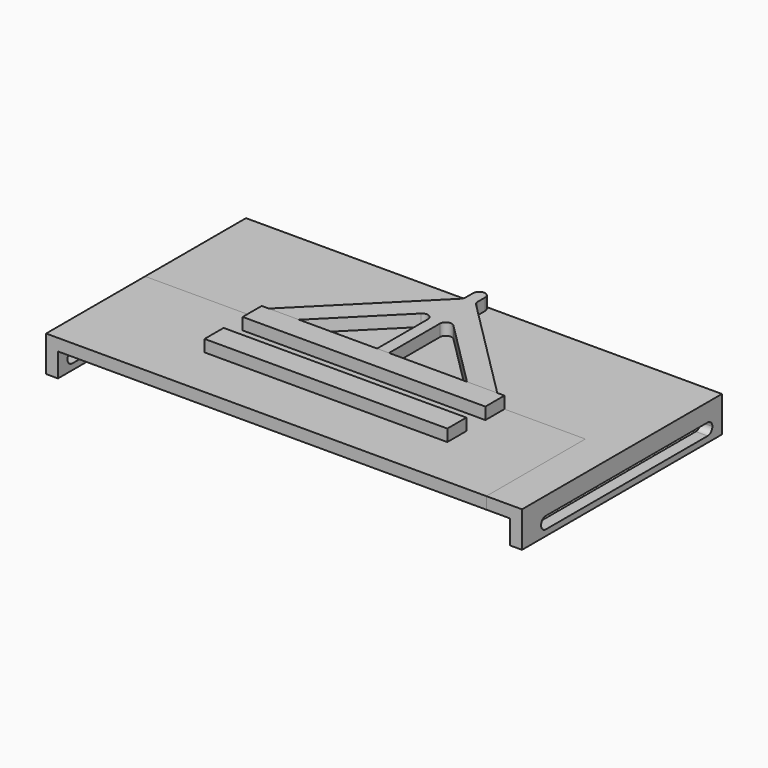
from build123d import *

# Parameters (mm, degrees)
F0_W      = 5
F0_H      = 53
F0_W_2    = 10
F0_H_2    = 10
F1_DEPTH  = 5
F2_DEPTH  = 10
F3_DEPTH  = 10
F0_W_3    = 48.5
F4_DEPTH  = 5
F5_DEPTH  = 10
F6_DEPTH  = 10
F8_DEPTH  = 25
F10_DEPTH = 25


with BuildPart() as f1:
    # F0 (on Top) → F1 (new body)
    with BuildSketch(Plane.XY):
        with Locations((97.5, 26)):
            Rectangle(F0_W, F0_H)
        with BuildLine():
            Line((0, 52.5), (-100, 52.5))
            Line((-100, 52.5), (-100, -0.5))
            Line((-100, -0.5), (-95, -0.5))
            Line((-95, -0.5), (-51, -0.5))
            Line((-51, -0.5), (-48, -0.5))
            Line((-48, -0.5), (-3.232233047, 44.267766953))
            ThreePointArc((-3.232233047, 44.267766953), (-2.6903011687, 45.078825325), (-2.5, 46.0355339059))
            Line((-2.5, 46.0355339059), (-2.5, 50))
            ThreePointArc((-2.5, 50), (-1.767766953, 51.767766953), (0, 52.5))
        make_face()
        with BuildLine():
            Line((85, 52.5), (0, 52.5))
            ThreePointArc((0, 52.5), (1.767766953, 51.767766953), (2.5, 50))
            Line((2.5, 50), (2.5, 46.0355339059))
            ThreePointArc((2.5, 46.0355339059), (2.6903011687, 45.078825325), (3.232233047, 44.267766953))
            Line((3.232233047, 44.267766953), (48, -0.5))
            Line((48, -0.5), (51, -0.5))
            Line((51, -0.5), (85, -0.5))
            Line((85, -0.5), (85, 52.5))
        make_face()
        with BuildLine():
            ThreePointArc((2.5, 50), (1.767766953, 51.767766953), (0, 52.5))
            ThreePointArc((0, 52.5), (-1.767766953, 51.767766953), (-2.5, 50))
            Line((-2.5, 50), (-2.5, 46.0355339059))
            Line((-2.5, 46.0355339059), (-2.5, 32.2720779386))
            Line((-2.5, 32.2720779386), (-2.5, 26.2365440327))
            Line((-2.5, 26.2365440327), (-2.5, 0))
            Line((-2.5, 0), (-2.5, -0.5))
            Line((-2.5, -0.5), (2.5, -0.5))
            Line((2.5, -0.5), (2.5, 26.2365440327))
            Line((2.5, 26.2365440327), (2.5, 46.0355339059))
            Line((2.5, 46.0355339059), (2.5, 50))
        make_face()
        with BuildLine():
            Line((-2.5, 32.2720779386), (-2.5, 46.0355339059))
            ThreePointArc((-2.5, 46.0355339059), (-2.6903011687, 45.078825325), (-3.232233047, 44.267766953))
            Line((-3.232233047, 44.267766953), (-48, -0.5))
            Line((-48, -0.5), (-35.2720779386, -0.5))
            Line((-35.2720779386, -0.5), (-6.767766953, 28.0043109857))
            ThreePointArc((-6.767766953, 28.0043109857), (-4.0432914191, 28.546242864), (-2.5, 26.2365440327))
            Line((-2.5, 26.2365440327), (-2.5, 32.2720779386))
        make_face()
        with BuildLine():
            Line((-2.5, 0), (-2.5, 26.2365440327))
            ThreePointArc((-2.5, 26.2365440327), (-4.0432914191, 28.546242864), (-6.767766953, 28.0043109857))
            Line((-6.767766953, 28.0043109857), (-35.2720779386, -0.5))
            Line((-35.2720779386, -0.5), (-2.5, -0.5))
            Line((-2.5, -0.5), (-2.5, 0))
        make_face()
        with BuildLine():
            ThreePointArc((6.767766953, 28.0043109857), (4.0432914191, 28.546242864), (2.5, 26.2365440327))
            Line((2.5, 26.2365440327), (2.5, -0.5))
            Line((2.5, -0.5), (35.2720779386, -0.5))
            Line((35.2720779386, -0.5), (6.767766953, 28.0043109857))
        make_face()
        with BuildLine():
            ThreePointArc((3.232233047, 44.267766953), (2.6903011687, 45.078825325), (2.5, 46.0355339059))
            Line((2.5, 46.0355339059), (2.5, 26.2365440327))
            ThreePointArc((2.5, 26.2365440327), (4.0432914191, 28.546242864), (6.767766953, 28.0043109857))
            Line((6.767766953, 28.0043109857), (35.2720779386, -0.5))
            Line((35.2720779386, -0.5), (48, -0.5))
            Line((48, -0.5), (3.232233047, 44.267766953))
        make_face()
        with Locations((90, 26)):
            Rectangle(F0_W_2, F0_H)
        with Locations((90, -5.5)):
            Rectangle(F0_W_2, F0_H_2)
        with Locations((90, -15.5)):
            Rectangle(F0_W_2, F0_H_2)
        with Locations((90, -25.5)):
            Rectangle(F0_W_2, F0_H_2)
        with Locations((97.5, -25.5)):
            Rectangle(F0_W, F0_H_2)
        with Locations((97.5, -15.5)):
            Rectangle(F0_W, F0_H_2)
        with Locations((97.5, -5.5)):
            Rectangle(F0_W, F0_H_2)
        Polygon((95, -30.5), (85, -30.5), (85, -37.5), (95, -47.5), align=None)
        with BuildLine():
            Line((100, -30.5), (95, -30.5))
            Line((95, -30.5), (95, -47.5))
            Line((95, -47.5), (95.732233047, -48.232233047))
            ThreePointArc((95.732233047, -48.232233047), (96.4244505146, -50.4455071839), (95, -52.2754493028))
            Line((95, -52.2754493028), (95, -52.5))
            Line((95, -52.5), (100, -52.5))
            Line((100, -52.5), (100, -30.5))
        make_face()
        with BuildLine():
            Line((95, -47.5), (85, -37.5))
            Line((85, -37.5), (85, -50.2279220614))
            Line((85, -50.2279220614), (86.5398448916, -51.767766953))
            ThreePointArc((86.5398448916, -51.767766953), (87.3509032637, -52.3096988313), (88.3076118446, -52.5))
            Line((88.3076118446, -52.5), (93.9644660941, -52.5))
            ThreePointArc((93.9644660941, -52.5), (94.4942664069, -52.4432174747), (95, -52.2754493028))
            Line((95, -52.2754493028), (95, -47.5))
        make_face()
        with BuildLine():
            Line((86.5398448916, -51.767766953), (85, -50.2279220614))
            Line((85, -50.2279220614), (85, -52.5))
            Line((85, -52.5), (88.3076118446, -52.5))
            ThreePointArc((88.3076118446, -52.5), (87.3509032637, -52.3096988313), (86.5398448916, -51.767766953))
        make_face()
        with BuildLine():
            Line((95.732233047, -48.232233047), (95, -47.5))
            Line((95, -47.5), (95, -52.2754493028))
            ThreePointArc((95, -52.2754493028), (96.4244505146, -50.4455071839), (95.732233047, -48.232233047))
        make_face()
        with BuildLine():
            Line((95, -52.5), (95, -52.2754493028))
            ThreePointArc((95, -52.2754493028), (94.4942664069, -52.4432174747), (93.9644660941, -52.5))
            Line((93.9644660941, -52.5), (95, -52.5))
        make_face()
    extrude(amount=F1_DEPTH)

    # F0 (on Top) → F2 (join)
    with BuildSketch(Plane.XY):
        with BuildLine():
            ThreePointArc((2.5, 50), (1.767766953, 51.767766953), (0, 52.5))
            ThreePointArc((0, 52.5), (-1.767766953, 51.767766953), (-2.5, 50))
            Line((-2.5, 50), (-2.5, 46.0355339059))
            Line((-2.5, 46.0355339059), (-2.5, 32.2720779386))
            Line((-2.5, 32.2720779386), (-2.5, 26.2365440327))
            Line((-2.5, 26.2365440327), (-2.5, 0))
            Line((-2.5, 0), (-2.5, -0.5))
            Line((-2.5, -0.5), (2.5, -0.5))
            Line((2.5, -0.5), (2.5, 26.2365440327))
            Line((2.5, 26.2365440327), (2.5, 46.0355339059))
            Line((2.5, 46.0355339059), (2.5, 50))
        make_face()
        with BuildLine():
            Line((-2.5, 32.2720779386), (-2.5, 46.0355339059))
            ThreePointArc((-2.5, 46.0355339059), (-2.6903011687, 45.078825325), (-3.232233047, 44.267766953))
            Line((-3.232233047, 44.267766953), (-48, -0.5))
            Line((-48, -0.5), (-35.2720779386, -0.5))
            Line((-35.2720779386, -0.5), (-6.767766953, 28.0043109857))
            ThreePointArc((-6.767766953, 28.0043109857), (-4.0432914191, 28.546242864), (-2.5, 26.2365440327))
            Line((-2.5, 26.2365440327), (-2.5, 32.2720779386))
        make_face()
        with BuildLine():
            ThreePointArc((3.232233047, 44.267766953), (2.6903011687, 45.078825325), (2.5, 46.0355339059))
            Line((2.5, 46.0355339059), (2.5, 26.2365440327))
            ThreePointArc((2.5, 26.2365440327), (4.0432914191, 28.546242864), (6.767766953, 28.0043109857))
            Line((6.767766953, 28.0043109857), (35.2720779386, -0.5))
            Line((35.2720779386, -0.5), (48, -0.5))
            Line((48, -0.5), (3.232233047, 44.267766953))
        make_face()
    extrude(amount=F2_DEPTH)

    # F0 (on Top) → F3 (join)
    with BuildSketch(Plane.XY):
        with Locations((97.5, 26)):
            Rectangle(F0_W, F0_H)
        with Locations((97.5, -5.5)):
            Rectangle(F0_W, F0_H_2)
        with Locations((97.5, -15.5)):
            Rectangle(F0_W, F0_H_2)
        with Locations((97.5, -25.5)):
            Rectangle(F0_W, F0_H_2)
        with BuildLine():
            Line((100, -30.5), (95, -30.5))
            Line((95, -30.5), (95, -47.5))
            Line((95, -47.5), (95.732233047, -48.232233047))
            ThreePointArc((95.732233047, -48.232233047), (96.4244505146, -50.4455071839), (95, -52.2754493028))
            Line((95, -52.2754493028), (95, -52.5))
            Line((95, -52.5), (100, -52.5))
            Line((100, -52.5), (100, -30.5))
        make_face()
        with BuildLine():
            Line((95.732233047, -48.232233047), (95, -47.5))
            Line((95, -47.5), (95, -52.2754493028))
            ThreePointArc((95, -52.2754493028), (96.4244505146, -50.4455071839), (95.732233047, -48.232233047))
        make_face()
    extrude(amount=-F3_DEPTH)

    # F7 (on face) → F8 (cut)
    with BuildSketch(Plane.YZ.offset(100)):
        with BuildLine():
            Line((45, -2.5), (-40, -2.5))
            ThreePointArc((-40, -2.5), (-41.767766953, -3.232233047), (-42.5, -5))
            ThreePointArc((-42.5, -5), (-41.767766953, -6.767766953), (-40, -7.5))
            Line((-40, -7.5), (45, -7.5))
            ThreePointArc((45, -7.5), (46.767766953, -6.767766953), (47.5, -5))
            ThreePointArc((47.5, -5), (46.767766953, -3.232233047), (45, -2.5))
        make_face()
    extrude(amount=-F8_DEPTH, mode=Mode.SUBTRACT)


with BuildPart() as f4:
    # F0 (on Top) → F4 (new body)
    with BuildSketch(Plane.XY):
        with Locations((-97.5, -25.5)):
            Rectangle(F0_W, F0_H_2)
        Polygon((-68, -20.5), (-95, -20.5), (-95, -30.5), (-78, -30.5), align=None)
        with Locations((-97.5, -15.5)):
            Rectangle(F0_W, F0_H_2)
        with Locations((-97.5, -5.5)):
            Rectangle(F0_W, F0_H_2)
        Polygon((-51, -0.5), (-95, -0.5), (-95, -10.5), (-58, -10.5), (-51, -3.5), align=None)
        Polygon((-58, -10.5), (-95, -10.5), (-95, -20.5), (-68, -20.5), align=None)
        Polygon((-55.2720779386, -20.5), (-68, -20.5), (-78, -30.5), (-65.2720779386, -30.5), align=None)
        Polygon((-51, -10.5), (-58, -10.5), (-68, -20.5), (-55.2720779386, -20.5), (-45.2720779386, -10.5), align=None)
        Polygon((-35.2720779386, -0.5), (-48, -0.5), (-51, -3.5), (-51, -10.5), (-45.2720779386, -10.5), align=None)
        Polygon((-51, -3.5), (-58, -10.5), (-51, -10.5), align=None)
        Polygon((-48, -0.5), (-51, -0.5), (-51, -3.5), align=None)
        Polygon((-2.5, -0.5), (-35.2720779386, -0.5), (-45.2720779386, -10.5), (-2.5, -10.5), align=None)
        Polygon((-45.2720779386, -10.5), (-55.2720779386, -20.5), (-51, -20.5), (-2.5, -20.5), (-2.5, -10.5), align=None)
        Polygon((-51, -20.5), (-55.2720779386, -20.5), (-65.2720779386, -30.5), (-51, -30.5), align=None)
        with Locations((-26.75, -25.5)):
            Rectangle(F0_W_3, F0_H_2)
        with Locations((0, -5.5)):
            Rectangle(F0_W, F0_H_2)
        with Locations((0, -15.5)):
            Rectangle(F0_W, F0_H_2)
        with Locations((0, -25.5)):
            Rectangle(F0_W, F0_H_2)
        Polygon((45.2720779386, -10.5), (2.5, -10.5), (2.5, -20.5), (51, -20.5), (55.2720779386, -20.5), align=None)
        Polygon((35.2720779386, -0.5), (2.5, -0.5), (2.5, -10.5), (45.2720779386, -10.5), align=None)
        Polygon((65.2720779386, -30.5), (55.2720779386, -20.5), (51, -20.5), (51, -30.5), align=None)
        Polygon((78, -30.5), (68, -20.5), (55.2720779386, -20.5), (65.2720779386, -30.5), align=None)
        Polygon((68, -20.5), (58, -10.5), (51, -10.5), (45.2720779386, -10.5), (55.2720779386, -20.5), align=None)
        with Locations((26.75, -25.5)):
            Rectangle(F0_W_3, F0_H_2)
        Polygon((51, -3.5), (48, -0.5), (35.2720779386, -0.5), (45.2720779386, -10.5), (51, -10.5), align=None)
        Polygon((51, -3.5), (51, -0.5), (48, -0.5), align=None)
        Polygon((58, -10.5), (51, -3.5), (51, -10.5), align=None)
        Polygon((85, -30.5), (85, -20.5), (68, -20.5), (78, -30.5), align=None)
        Polygon((85, -20.5), (85, -10.5), (58, -10.5), (68, -20.5), align=None)
        Polygon((85, -10.5), (85, -0.5), (51, -0.5), (51, -3.5), (58, -10.5), align=None)
        Polygon((85, -37.5), (85, -30.5), (78, -30.5), align=None)
        Polygon((85, -37.5), (78, -30.5), (65.2720779386, -30.5), (85, -50.2279220614), align=None)
        with BuildLine():
            Line((85, -50.2279220614), (65.2720779386, -30.5))
            Line((65.2720779386, -30.5), (51, -30.5))
            Line((51, -30.5), (2.5, -30.5))
            Line((2.5, -30.5), (2.5, -50))
            ThreePointArc((2.5, -50), (1.767766953, -51.767766953), (0, -52.5))
            Line((0, -52.5), (85, -52.5))
            Line((85, -52.5), (85, -50.2279220614))
        make_face()
        with BuildLine():
            Line((2.5, -50), (2.5, -30.5))
            Line((2.5, -30.5), (-2.5, -30.5))
            Line((-2.5, -30.5), (-2.5, -50))
            ThreePointArc((-2.5, -50), (-1.767766953, -51.767766953), (0, -52.5))
            ThreePointArc((0, -52.5), (1.767766953, -51.767766953), (2.5, -50))
        make_face()
        with BuildLine():
            Line((-51, -30.5), (-65.2720779386, -30.5))
            Line((-65.2720779386, -30.5), (-86.5398448916, -51.767766953))
            ThreePointArc((-86.5398448916, -51.767766953), (-87.3509032637, -52.3096988313), (-88.3076118446, -52.5))
            Line((-88.3076118446, -52.5), (0, -52.5))
            ThreePointArc((0, -52.5), (-1.767766953, -51.767766953), (-2.5, -50))
            Line((-2.5, -50), (-2.5, -30.5))
            Line((-2.5, -30.5), (-51, -30.5))
        make_face()
        with BuildLine():
            Line((-65.2720779386, -30.5), (-78, -30.5))
            Line((-78, -30.5), (-95, -47.5))
            Line((-95, -47.5), (-95, -52.2754493028))
            ThreePointArc((-95, -52.2754493028), (-94.4942664069, -52.4432174747), (-93.9644660941, -52.5))
            Line((-93.9644660941, -52.5), (-88.3076118446, -52.5))
            ThreePointArc((-88.3076118446, -52.5), (-87.3509032637, -52.3096988313), (-86.5398448916, -51.767766953))
            Line((-86.5398448916, -51.767766953), (-65.2720779386, -30.5))
        make_face()
        with BuildLine():
            Line((-95, -30.5), (-100, -30.5))
            Line((-100, -30.5), (-100, -52.5))
            Line((-100, -52.5), (-95, -52.5))
            Line((-95, -52.5), (-95, -52.2754493028))
            ThreePointArc((-95, -52.2754493028), (-96.4244505146, -50.4455071839), (-95.732233047, -48.232233047))
            Line((-95.732233047, -48.232233047), (-95, -47.5))
            Line((-95, -47.5), (-95, -30.5))
        make_face()
        with BuildLine():
            Line((-95, -52.2754493028), (-95, -52.5))
            Line((-95, -52.5), (-93.9644660941, -52.5))
            ThreePointArc((-93.9644660941, -52.5), (-94.4942664069, -52.4432174747), (-95, -52.2754493028))
        make_face()
        Polygon((-78, -30.5), (-95, -30.5), (-95, -47.5), align=None)
        with BuildLine():
            Line((-95, -52.2754493028), (-95, -47.5))
            Line((-95, -47.5), (-95.732233047, -48.232233047))
            ThreePointArc((-95.732233047, -48.232233047), (-96.4244505146, -50.4455071839), (-95, -52.2754493028))
        make_face()
    extrude(amount=F4_DEPTH)

    # F0 (on Top) → F5 (join)
    with BuildSketch(Plane.XY):
        with Locations((-97.5, -5.5)):
            Rectangle(F0_W, F0_H_2)
        with Locations((-97.5, -15.5)):
            Rectangle(F0_W, F0_H_2)
        with Locations((-97.5, -25.5)):
            Rectangle(F0_W, F0_H_2)
        with BuildLine():
            Line((-95, -30.5), (-100, -30.5))
            Line((-100, -30.5), (-100, -52.5))
            Line((-100, -52.5), (-95, -52.5))
            Line((-95, -52.5), (-95, -52.2754493028))
            ThreePointArc((-95, -52.2754493028), (-96.4244505146, -50.4455071839), (-95.732233047, -48.232233047))
            Line((-95.732233047, -48.232233047), (-95, -47.5))
            Line((-95, -47.5), (-95, -30.5))
        make_face()
        with BuildLine():
            Line((-95, -52.2754493028), (-95, -47.5))
            Line((-95, -47.5), (-95.732233047, -48.232233047))
            ThreePointArc((-95.732233047, -48.232233047), (-96.4244505146, -50.4455071839), (-95, -52.2754493028))
        make_face()
    extrude(amount=-F5_DEPTH)

    # F0 (on Top) → F6 (join)
    with BuildSketch(Plane.XY):
        Polygon((-2.5, -0.5), (-35.2720779386, -0.5), (-45.2720779386, -10.5), (-2.5, -10.5), align=None)
        Polygon((-35.2720779386, -0.5), (-48, -0.5), (-51, -3.5), (-51, -10.5), (-45.2720779386, -10.5), align=None)
        Polygon((-48, -0.5), (-51, -0.5), (-51, -3.5), align=None)
        with Locations((-26.75, -25.5)):
            Rectangle(F0_W_3, F0_H_2)
        with Locations((26.75, -25.5)):
            Rectangle(F0_W_3, F0_H_2)
        with Locations((0, -25.5)):
            Rectangle(F0_W, F0_H_2)
        Polygon((35.2720779386, -0.5), (2.5, -0.5), (2.5, -10.5), (45.2720779386, -10.5), align=None)
        with Locations((0, -5.5)):
            Rectangle(F0_W, F0_H_2)
        Polygon((51, -3.5), (48, -0.5), (35.2720779386, -0.5), (45.2720779386, -10.5), (51, -10.5), align=None)
        Polygon((51, -3.5), (51, -0.5), (48, -0.5), align=None)
    extrude(amount=F6_DEPTH)

    # F9 (on face) → F10 (cut)
    with BuildSketch(Plane(origin=(-100, 0, 0), x_dir=(0, -1, 0), z_dir=(-1, 0, 0))):
        with BuildLine():
            Line((45, -2.5), (10, -2.5))
            ThreePointArc((10, -2.5), (8.232233047, -3.232233047), (7.5, -5))
            ThreePointArc((7.5, -5), (8.232233047, -6.767766953), (10, -7.5))
            Line((10, -7.5), (45, -7.5))
            ThreePointArc((45, -7.5), (46.767766953, -6.767766953), (47.5, -5))
            ThreePointArc((47.5, -5), (46.767766953, -3.232233047), (45, -2.5))
        make_face()
    extrude(amount=-F10_DEPTH, mode=Mode.SUBTRACT)


solid = Compound([f1.part, f4.part])
